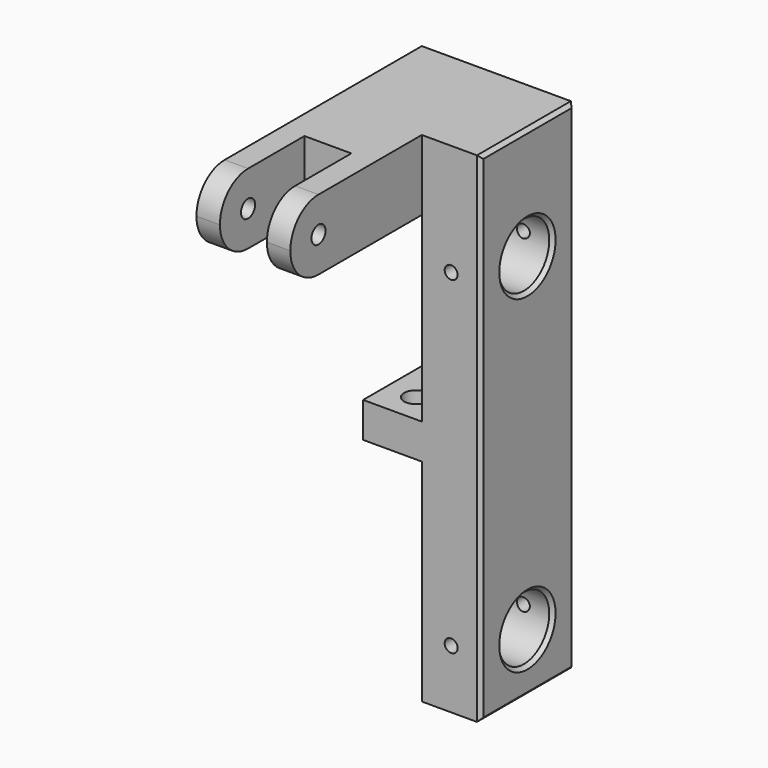
from build123d import *

# Parameters (mm, degrees)
F0_W     = 4
F0_H     = 6
F1_DEPTH = 15
F0_W_2   = 2
F2_DEPTH = 24
F0_W_3   = 5
F3_DEPTH = 10
F4_R     = 2.99999
F5_R     = 2.7
F5_R_2   = 0.75
F6_DEPTH = 13.001
F7_D     = 1.1
F7_DEPTH = 40
F7_TIP   = 0.3304733405
F8_R     = 1
F9_DEPTH = 21.001
F10_SIZE = 0.3


# Not quite as in the source:
# - a fillet or chamfer is up to 0.001 mm smaller than in the source, because OpenCascade refuses the exact size


with BuildPart() as f1:
    # F0 (on Front) → F1 (new body)
    with BuildSketch(Plane.XZ):
        with Locations((-9, 39.5)):
            Rectangle(F0_W, F0_H)
    extrude(amount=F1_DEPTH)

    # F0 (on Front) → F2 (join)
    with BuildSketch(Plane.XZ):
        with Locations((-12, 39.5)):
            Rectangle(F0_W_2, F0_H)
        with Locations((-6, 39.5)):
            Rectangle(F0_W_2, F0_H)
    extrude(amount=F2_DEPTH)

    # F0 (on Front) → F3 (join)
    with BuildSketch(Plane.XZ):
        with Locations((-2.5, 39.5)):
            Rectangle(F0_W_3, F0_H)
        Polygon((0, 36.5), (-5, 36.5), (-5, 21), (-10, 21), (-10, 18), (-5, 18), (-5, 0), (0, 0), align=None)
    extrude(amount=F3_DEPTH)

    # F4 (radius 3 in the source; OpenCascade refuses exactly that, so slightly less here)
    f4_edges = [f1.edges().sort_by_distance(p)[0] for p in [
        (-6, -24, 42.5),
        (-6, -24, 36.5),
        (-12, -24, 42.5),
        (-12, -24, 36.5),
    ]]
    fillet(f4_edges, radius=F4_R)

    # F5 (on face) → F6 (cut, through all)
    with BuildSketch(Plane(origin=(-13, 0, 0), x_dir=(0, -1, 0), z_dir=(-1, 0, 0))):
        with Locations((5, 33)):
            Circle(F5_R)
        with Locations((5, 5)):
            Circle(F5_R)
        with Locations((21, 39.5)):
            Circle(F5_R_2)
    extrude(amount=-F6_DEPTH, mode=Mode.SUBTRACT)

    # F7
    with Locations(Plane(origin=(0, 0, 0), x_dir=(1, 0, 0), z_dir=(0, 1, 0))):
        with Locations((-2.5, -33), (-2.5, -5)):
            Hole(F7_D / 2, depth=F7_DEPTH)
            with Locations((0, 0, -(F7_DEPTH + F7_TIP / 2))):  # 118° drill point
                Cone(0, F7_D / 2, F7_TIP, mode=Mode.SUBTRACT)

    # F8 (on face) → F9 (cut, through all)
    with BuildSketch(Plane.XY.offset(21)):
        with Locations((-7.5, -7.5)):
            Circle(F8_R)
    extrude(amount=-F9_DEPTH, mode=Mode.SUBTRACT)

    # F10
    f10_edges = [f1.edges().sort_by_distance(p)[0] for p in [
        (0, -5, 0),
        (0, 0, 21.25),
        (0, -10, 21.25),
        (0, -5, 42.5),
        (0, -2.3, 5),
        (0, -2.3, 33),
    ]]
    chamfer(f10_edges, length=F10_SIZE)


solid = f1.part
